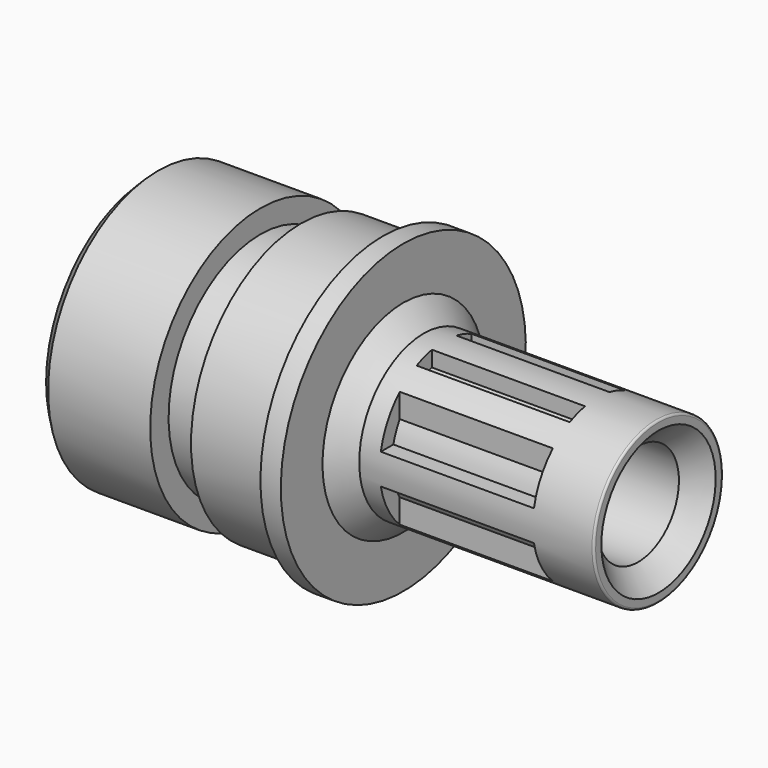
from build123d import *

# Parameters (mm, degrees)
F2_R             = 0.2
F3_SIZE          = 2
F4_SIZE          = 1
F7_DEPTH         = 15
F7_COPIES2_COUNT = 2


# Not quite as in the source:
# - a pattern or mirror of a feature is missing from the dataset's text; its kind, count and spacing are read off the source's solid


with BuildPart() as f1:
    # F0 (on Front) → F1 (revolve)
    with BuildSketch(Plane.XZ):
        Polygon((0, 13.5), (0, 11), (22, 5), (50, 5), (50, 7.9), (25, 7.9), (25, 15), (23, 15), (23, 13.5), (15, 13.5), (15, 11.25), (11, 11.25), (11, 13.5), align=None)
    revolve(axis=Axis((18.4335876124, 0, 0), (-1, 0, 0)))

    # F2
    f2_edges = [f1.edges().sort_by_distance(p)[0] for p in [
        (50, 0, -7.9),
    ]]
    fillet(f2_edges, radius=F2_R)

    # F3
    f3_edges = [f1.edges().sort_by_distance(p)[0] for p in [
        (50, 0, -5),
        (25, 0, -7.9),
    ]]
    chamfer(f3_edges, length=F3_SIZE)

    # F4
    f4_edges = [f1.edges().sort_by_distance(p)[0] for p in [
        (0, 0, -13.5),
    ]]
    chamfer(f4_edges, length=F4_SIZE)

    # F6 (on offset) → F7 (cut)
    with BuildSketch(Plane.YZ.offset(44)):
        with BuildLine():
            ThreePointArc((-3.37, 5.4408730917), (-2.4661025438, 5.905788537), (-1.5, 6.2217360921))
            Line((-1.5, 6.2217360921), (-1.5, 7.7562877719))
            ThreePointArc((-1.5, 7.7562877719), (-2.4540983699, 7.5091544924), (-3.37, 7.145145205))
            Line((-3.37, 7.145145205), (-3.37, 5.4408730917))
        make_face()
        with BuildLine():
            Line((-5.44, 3.3714092009), (-5.44, 5.7285600285))
            ThreePointArc((-5.44, 5.7285600285), (-6.928613333, 3.7953020014), (-7.7562877719, 1.5))
            Line((-7.7562877719, 1.5), (-6.2217360921, 1.5))
            ThreePointArc((-6.2217360921, 1.5), (-5.9054690982, 2.4668673921), (-5.44, 3.3714092009))
        make_face()
    f7 = extrude(amount=-F7_DEPTH, mode=Mode.SUBTRACT)

    # F7_copies: F7 across plane
    add(f7.mirror(Plane.ZX), mode=Mode.SUBTRACT)

    # F7_copies1: F7 across plane
    add(f7.mirror(Plane(origin=(0, 0, 0), x_dir=(-1, 0, 0), z_dir=(0, 0, -1))), mode=Mode.SUBTRACT)

    # F7_copies2: F7 ×2 about axis
    f7_copies2_axis = Axis((0, 0, 0), (1, 0, 0))
    for i in range(1, F7_COPIES2_COUNT):
        add(f7.rotate(f7_copies2_axis, i * 360 / F7_COPIES2_COUNT), mode=Mode.SUBTRACT)


solid = f1.part
